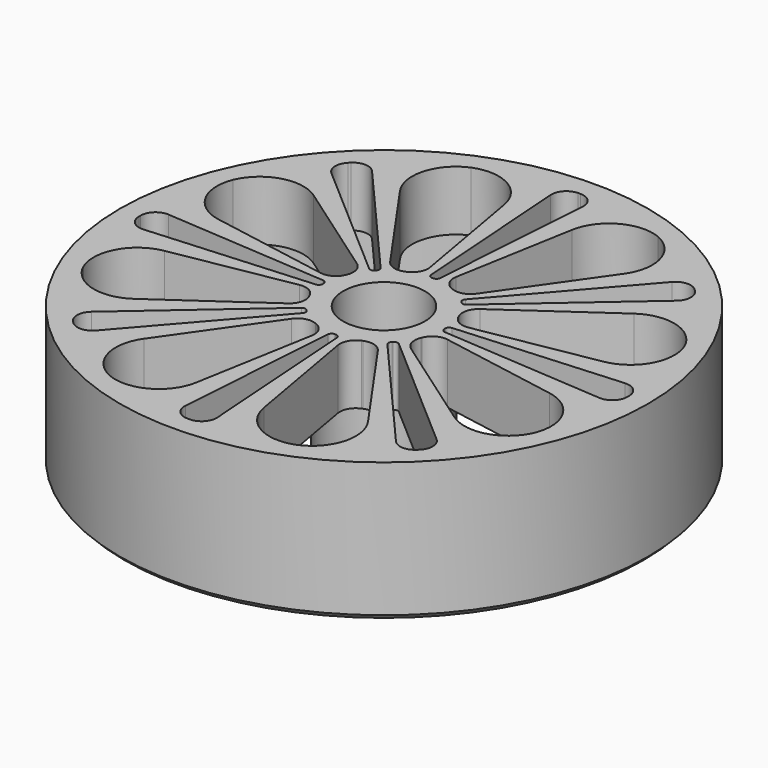
from build123d import *

# Parameters (mm, degrees)
F0_R        = 26.5
F0_R_2      = 4.1
F1_DEPTH    = 6
F3_DEPTH    = 6
F4_R        = 0.4
F5_R        = 1.6
F6_R        = 1.5
F7_T1_DEPTH = 6
F8_R        = 26.5
F8_R_2      = 24.9
F8_R_3      = 5.7
F8_R_4      = 4.1
F9_DEPTH    = 8
F10_SIZE    = 0.5


# Not quite as in the source:
# - a fillet or chamfer that OpenCascade refuses, or shapes differently, is made with other operations: its cross-section is extruded or revolved along the edge and cut away or added


with BuildPart() as f1:
    # F0 (on Top) → F1 (new body)
    with BuildSketch(Plane.XY):
        Circle(F0_R)
        Circle(F0_R_2, mode=Mode.SUBTRACT)
    extrude(amount=F1_DEPTH)

    # F2 (on face) → F3 (cut, through all)
    with BuildSketch(Plane(origin=(0, 0, 0), x_dir=(1, 0, 0), z_dir=(0, 0, -1))):
        with BuildLine():
            ThreePointArc((4.9968274702, 3.4988162617), (5.6356651483, 2.3343689374), (6.0073272934, 1.0592538838))
            Line((6.0073272934, 1.0592538838), (24.1277899488, 4.2543803528))
            ThreePointArc((24.1277899488, 4.2543803528), (22.6350485465, 9.3757440929), (20.0692250851, 14.0526226906))
            Line((20.0692250851, 14.0526226906), (4.9968274702, 3.4988162617))
        make_face()
        with BuildLine():
            ThreePointArc((6.0851407066, 0.4255144898), (6.0962840448, 0.2128869299), (6.1, 0))
            ThreePointArc((6.1, 0), (6.0962840448, -0.2128869299), (6.0851407066, -0.4255144898))
            Line((6.0851407066, -0.4255144898), (24.4403192314, -1.7090336067))
            ThreePointArc((24.4403192314, -1.7090336067), (24.485075262, -0.8550376692), (24.5, 0))
            ThreePointArc((24.5, 0), (24.485075262, 0.8550376692), (24.4403192314, 1.7090336067))
            Line((24.4403192314, 1.7090336067), (6.0851407066, 0.4255144898))
        make_face()
        with BuildLine():
            Line((24.1277899488, -4.2543803528), (6.0073272934, -1.0592538838))
            ThreePointArc((6.0073272934, -1.0592538838), (5.6356651483, -2.3343689374), (4.9968274702, -3.4988162617))
            Line((4.9968274702, -3.4988162617), (20.0692250851, -14.0526226906))
            ThreePointArc((20.0692250851, -14.0526226906), (22.6350485465, -9.3757440929), (24.1277899488, -4.2543803528))
        make_face()
        with BuildLine():
            Line((18.4903847155, -16.0734462103), (4.6037284394, -4.0019600768))
            ThreePointArc((4.6037284394, -4.0019600768), (4.3133513652, -4.3133513652), (4.0019600768, -4.6037284394))
            Line((4.0019600768, -4.6037284394), (16.0734462103, -18.4903847155))
            ThreePointArc((16.0734462103, -18.4903847155), (17.3241161391, -17.3241161391), (18.4903847155, -16.0734462103))
        make_face()
        with BuildLine():
            Line((14.0526226906, -20.0692250851), (3.4988162617, -4.9968274702))
            ThreePointArc((3.4988162617, -4.9968274702), (2.3343689374, -5.6356651483), (1.0592538838, -6.0073272934))
            Line((1.0592538838, -6.0073272934), (4.2543803528, -24.1277899488))
            ThreePointArc((4.2543803528, -24.1277899488), (9.3757440929, -22.6350485465), (14.0526226906, -20.0692250851))
        make_face()
        with BuildLine():
            Line((1.7090336067, -24.4403192314), (0.4255144898, -6.0851407066))
            ThreePointArc((0.4255144898, -6.0851407066), (0, -6.1), (-0.4255144898, -6.0851407066))
            Line((-0.4255144898, -6.0851407066), (-1.7090336067, -24.4403192314))
            ThreePointArc((-1.7090336067, -24.4403192314), (0, -24.5), (1.7090336067, -24.4403192314))
        make_face()
        with BuildLine():
            Line((-4.2543803528, -24.1277899488), (-1.0592538838, -6.0073272934))
            ThreePointArc((-1.0592538838, -6.0073272934), (-2.3343689374, -5.6356651483), (-3.4988162617, -4.9968274702))
            Line((-3.4988162617, -4.9968274702), (-14.0526226906, -20.0692250851))
            ThreePointArc((-14.0526226906, -20.0692250851), (-9.3757440929, -22.6350485465), (-4.2543803528, -24.1277899488))
        make_face()
        with BuildLine():
            Line((-16.0734462103, -18.4903847155), (-4.0019600768, -4.6037284394))
            ThreePointArc((-4.0019600768, -4.6037284394), (-4.3133513652, -4.3133513652), (-4.6037284394, -4.0019600768))
            Line((-4.6037284394, -4.0019600768), (-18.4903847155, -16.0734462103))
            ThreePointArc((-18.4903847155, -16.0734462103), (-17.3241161391, -17.3241161391), (-16.0734462103, -18.4903847155))
        make_face()
        with BuildLine():
            Line((-20.0692250851, -14.0526226906), (-4.9968274702, -3.4988162617))
            ThreePointArc((-4.9968274702, -3.4988162617), (-5.6356651483, -2.3343689374), (-6.0073272934, -1.0592538838))
            Line((-6.0073272934, -1.0592538838), (-24.1277899488, -4.2543803528))
            ThreePointArc((-24.1277899488, -4.2543803528), (-22.6350485465, -9.3757440929), (-20.0692250851, -14.0526226906))
        make_face()
        with BuildLine():
            ThreePointArc((-6.0851407066, -0.4255144898), (-6.1, 0), (-6.0851407066, 0.4255144898))
            Line((-6.0851407066, 0.4255144898), (-24.4403192314, 1.7090336067))
            ThreePointArc((-24.4403192314, 1.7090336067), (-24.5, 0), (-24.4403192314, -1.7090336067))
            Line((-24.4403192314, -1.7090336067), (-6.0851407066, -0.4255144898))
        make_face()
        with BuildLine():
            ThreePointArc((-6.0073272934, 1.0592538838), (-5.6356651483, 2.3343689374), (-4.9968274702, 3.4988162617))
            Line((-4.9968274702, 3.4988162617), (-20.0692250851, 14.0526226906))
            ThreePointArc((-20.0692250851, 14.0526226906), (-22.6350485465, 9.3757440929), (-24.1277899488, 4.2543803528))
            Line((-24.1277899488, 4.2543803528), (-6.0073272934, 1.0592538838))
        make_face()
        with BuildLine():
            ThreePointArc((-4.6037284394, 4.0019600768), (-4.3133513652, 4.3133513652), (-4.0019600768, 4.6037284394))
            Line((-4.0019600768, 4.6037284394), (-16.0734462103, 18.4903847155))
            ThreePointArc((-16.0734462103, 18.4903847155), (-17.3241161391, 17.3241161391), (-18.4903847155, 16.0734462103))
            Line((-18.4903847155, 16.0734462103), (-4.6037284394, 4.0019600768))
        make_face()
        with BuildLine():
            ThreePointArc((-3.4988162617, 4.9968274702), (-2.3343689374, 5.6356651483), (-1.0592538838, 6.0073272934))
            Line((-1.0592538838, 6.0073272934), (-4.2543803528, 24.1277899488))
            ThreePointArc((-4.2543803528, 24.1277899488), (-9.3757440929, 22.6350485465), (-14.0526226906, 20.0692250851))
            Line((-14.0526226906, 20.0692250851), (-3.4988162617, 4.9968274702))
        make_face()
        with BuildLine():
            ThreePointArc((-0.4255144898, 6.0851407066), (0, 6.1), (0.4255144898, 6.0851407066))
            Line((0.4255144898, 6.0851407066), (1.7090336067, 24.4403192314))
            ThreePointArc((1.7090336067, 24.4403192314), (0, 24.5), (-1.7090336067, 24.4403192314))
            Line((-1.7090336067, 24.4403192314), (-0.4255144898, 6.0851407066))
        make_face()
        with BuildLine():
            ThreePointArc((1.0592538838, 6.0073272934), (2.3343689374, 5.6356651483), (3.4988162617, 4.9968274702))
            Line((3.4988162617, 4.9968274702), (14.0526226906, 20.0692250851))
            ThreePointArc((14.0526226906, 20.0692250851), (9.3757440929, 22.6350485465), (4.2543803528, 24.1277899488))
            Line((4.2543803528, 24.1277899488), (1.0592538838, 6.0073272934))
        make_face()
        with BuildLine():
            ThreePointArc((4.0019600768, 4.6037284394), (4.3133513652, 4.3133513652), (4.6037284394, 4.0019600768))
            Line((4.6037284394, 4.0019600768), (18.4903847155, 16.0734462103))
            ThreePointArc((18.4903847155, 16.0734462103), (17.3241161391, 17.3241161391), (16.0734462103, 18.4903847155))
            Line((16.0734462103, 18.4903847155), (4.0019600768, 4.6037284394))
        make_face()
    extrude(amount=-F3_DEPTH, mode=Mode.SUBTRACT)

    # F4
    f4_edges = [f1.edges().sort_by_distance(p)[0] for p in [
        (-0.425514, -6.085141, 3),
        (0.425514, -6.085141, 3),
        (4.00196, -4.603728, 3),
        (4.603728, -4.00196, 3),
        (6.085141, -0.425514, 3),
        (6.085141, 0.425514, 3),
        (4.603728, 4.00196, 3),
        (4.00196, 4.603728, 3),
        (0.425514, 6.085141, 3),
        (-0.425514, 6.085141, 3),
        (-4.00196, 4.603728, 3),
        (-4.603728, 4.00196, 3),
        (-6.085141, -0.425514, 3),
        (-6.085141, 0.425514, 3),
        (-4.00196, -4.603728, 3),
        (-4.603728, -4.00196, 3),
    ]]
    fillet(f4_edges, radius=F4_R)

    # F5
    f5_edges = [f1.edges().sort_by_distance(p)[0] for p in [
        (-6.007327, 1.059254, 3),
        (-4.996827, 3.498816, 3),
        (-3.498816, 4.996827, 3),
        (-1.059254, 6.007327, 3),
        (1.059254, 6.007327, 3),
        (3.498816, 4.996827, 3),
        (4.996827, 3.498816, 3),
        (6.007327, 1.059254, 3),
        (6.007327, -1.059254, 3),
        (4.996827, -3.498816, 3),
        (3.498816, -4.996827, 3),
        (1.059254, -6.007327, 3),
        (-1.059254, -6.007327, 3),
        (-3.498816, -4.996827, 3),
        (-4.996827, -3.498816, 3),
        (-6.007327, -1.059254, 3),
    ]]
    fillet(f5_edges, radius=F5_R)

    # F6
    f6_edges = [f1.edges().sort_by_distance(p)[0] for p in [
        (16.073446, -18.490385, 3),
        (18.490385, -16.073446, 3),
        (24.440319, -1.709034, 3),
        (24.440319, 1.709034, 3),
        (18.490385, 16.073446, 3),
        (1.709034, 24.440319, 3),
        (16.073446, 18.490385, 3),
        (-1.709034, 24.440319, 3),
        (-16.073446, 18.490385, 3),
        (-18.490385, 16.073446, 3),
        (-24.440319, 1.709034, 3),
        (-24.440319, -1.709034, 3),
        (-16.073446, -18.490385, 3),
        (-18.490385, -16.073446, 3),
        (-1.709034, -24.440319, 3),
        (1.709034, -24.440319, 3),
    ]]
    fillet(f6_edges, radius=F6_R)

    # F7: fillet of radius 4.4 on 16 edges, made by hand

    # F7_s2 → F7_t1 (join)
    with BuildSketch(Plane.XY):
        with BuildLine():
            ThreePointArc((22.6112890899, 9.432900174), (22.410754213, 5.6273524023), (19.314538133, 3.4056741928))
            Line((19.314538133, 3.4056741928), (24.1277899488, 4.2543803528))
            ThreePointArc((24.1277899488, 4.2543803528), (23.5125422749, 6.8855178287), (22.6112890899, 9.432900174))
        make_face()
        with BuildLine():
            ThreePointArc((16.0656162056, 11.2492655731), (19.8259353192, 11.8676572317), (22.6586635261, 9.3185281675))
            ThreePointArc((22.6586635261, 9.3185281675), (21.4946744342, 11.7570817369), (20.0692250851, 14.0526226906))
            Line((20.0692250851, 14.0526226906), (16.0656162056, 11.2492655731))
        make_face()
        with BuildLine():
            ThreePointArc((9.3185281675, 22.6586635261), (11.8676572317, 19.8259353192), (11.2492655731, 16.0656162056))
            Line((11.2492655731, 16.0656162056), (14.0526226906, 20.0692250851))
            ThreePointArc((14.0526226906, 20.0692250851), (11.7570817369, 21.4946744342), (9.3185281675, 22.6586635261))
        make_face()
        with BuildLine():
            ThreePointArc((3.4056741928, 19.314538133), (5.6273524023, 22.410754213), (9.432900174, 22.6112890899))
            ThreePointArc((9.432900174, 22.6112890899), (6.8855178287, 23.5125422749), (4.2543803528, 24.1277899488))
            Line((4.2543803528, 24.1277899488), (3.4056741928, 19.314538133))
        make_face()
        with BuildLine():
            ThreePointArc((-9.432900174, 22.6112890899), (-5.6273524023, 22.410754213), (-3.4056741928, 19.314538133))
            Line((-3.4056741928, 19.314538133), (-4.2543803528, 24.1277899488))
            ThreePointArc((-4.2543803528, 24.1277899488), (-6.8855178287, 23.5125422749), (-9.432900174, 22.6112890899))
        make_face()
        with BuildLine():
            ThreePointArc((-11.2492655731, 16.0656162056), (-11.8676572317, 19.8259353192), (-9.3185281675, 22.6586635261))
            ThreePointArc((-9.3185281675, 22.6586635261), (-11.7570817369, 21.4946744342), (-14.0526226906, 20.0692250851))
            Line((-14.0526226906, 20.0692250851), (-11.2492655731, 16.0656162056))
        make_face()
        with BuildLine():
            ThreePointArc((-22.6586635261, 9.3185281675), (-19.8259353192, 11.8676572317), (-16.0656162056, 11.2492655731))
            Line((-16.0656162056, 11.2492655731), (-20.0692250851, 14.0526226906))
            ThreePointArc((-20.0692250851, 14.0526226906), (-21.4946744342, 11.7570817369), (-22.6586635261, 9.3185281675))
        make_face()
        with BuildLine():
            ThreePointArc((-19.314538133, 3.4056741928), (-22.410754213, 5.6273524023), (-22.6112890899, 9.432900174))
            ThreePointArc((-22.6112890899, 9.432900174), (-23.5125422749, 6.8855178287), (-24.1277899488, 4.2543803528))
            Line((-24.1277899488, 4.2543803528), (-19.314538133, 3.4056741928))
        make_face()
        with BuildLine():
            ThreePointArc((-22.6112890899, -9.432900174), (-22.410754213, -5.6273524023), (-19.314538133, -3.4056741928))
            Line((-19.314538133, -3.4056741928), (-24.1277899488, -4.2543803528))
            ThreePointArc((-24.1277899488, -4.2543803528), (-23.5125422749, -6.8855178287), (-22.6112890899, -9.432900174))
        make_face()
        with BuildLine():
            ThreePointArc((-16.0656162056, -11.2492655731), (-19.8259353192, -11.8676572317), (-22.6586635261, -9.3185281675))
            ThreePointArc((-22.6586635261, -9.3185281675), (-21.4946744342, -11.7570817369), (-20.0692250851, -14.0526226906))
            Line((-20.0692250851, -14.0526226906), (-16.0656162056, -11.2492655731))
        make_face()
        with BuildLine():
            ThreePointArc((-9.3185281675, -22.6586635261), (-11.8676572317, -19.8259353192), (-11.2492655731, -16.0656162056))
            Line((-11.2492655731, -16.0656162056), (-14.0526226906, -20.0692250851))
            ThreePointArc((-14.0526226906, -20.0692250851), (-11.7570817369, -21.4946744342), (-9.3185281675, -22.6586635261))
        make_face()
        with BuildLine():
            ThreePointArc((-3.4056741928, -19.314538133), (-5.6273524023, -22.410754213), (-9.432900174, -22.6112890899))
            ThreePointArc((-9.432900174, -22.6112890899), (-6.8855178287, -23.5125422749), (-4.2543803528, -24.1277899488))
            Line((-4.2543803528, -24.1277899488), (-3.4056741928, -19.314538133))
        make_face()
        with BuildLine():
            ThreePointArc((9.432900174, -22.6112890899), (5.6273524023, -22.410754213), (3.4056741928, -19.314538133))
            Line((3.4056741928, -19.314538133), (4.2543803528, -24.1277899488))
            ThreePointArc((4.2543803528, -24.1277899488), (6.8855178287, -23.5125422749), (9.432900174, -22.6112890899))
        make_face()
        with BuildLine():
            ThreePointArc((11.2492655731, -16.0656162056), (11.8676572317, -19.8259353192), (9.3185281675, -22.6586635261))
            ThreePointArc((9.3185281675, -22.6586635261), (11.7570817369, -21.4946744342), (14.0526226906, -20.0692250851))
            Line((14.0526226906, -20.0692250851), (11.2492655731, -16.0656162056))
        make_face()
        with BuildLine():
            ThreePointArc((22.6586635261, -9.3185281675), (19.8259353192, -11.8676572317), (16.0656162056, -11.2492655731))
            Line((16.0656162056, -11.2492655731), (20.0692250851, -14.0526226906))
            ThreePointArc((20.0692250851, -14.0526226906), (21.4946744342, -11.7570817369), (22.6586635261, -9.3185281675))
        make_face()
        with BuildLine():
            ThreePointArc((19.314538133, -3.4056741928), (22.410754213, -5.6273524023), (22.6112890899, -9.432900174))
            ThreePointArc((22.6112890899, -9.432900174), (23.5125422749, -6.8855178287), (24.1277899488, -4.2543803528))
            Line((24.1277899488, -4.2543803528), (19.314538133, -3.4056741928))
        make_face()
    extrude(amount=F7_T1_DEPTH)

    # F8 (on face) → F9 (join)
    with BuildSketch(Plane(origin=(0, 0, 0), x_dir=(1, 0, 0), z_dir=(0, 0, -1))):
        Circle(F8_R)
        Circle(F8_R_2, mode=Mode.SUBTRACT)
        Circle(F8_R_3)
        Circle(F8_R_4, mode=Mode.SUBTRACT)
    extrude(amount=F9_DEPTH)

    # F10
    f10_edges = [f1.edges().sort_by_distance(p)[0] for p in [
        (-26.5, 0, -8),
        (-4.1, 0, -8),
    ]]
    chamfer(f10_edges, length=F10_SIZE)


solid = f1.part
